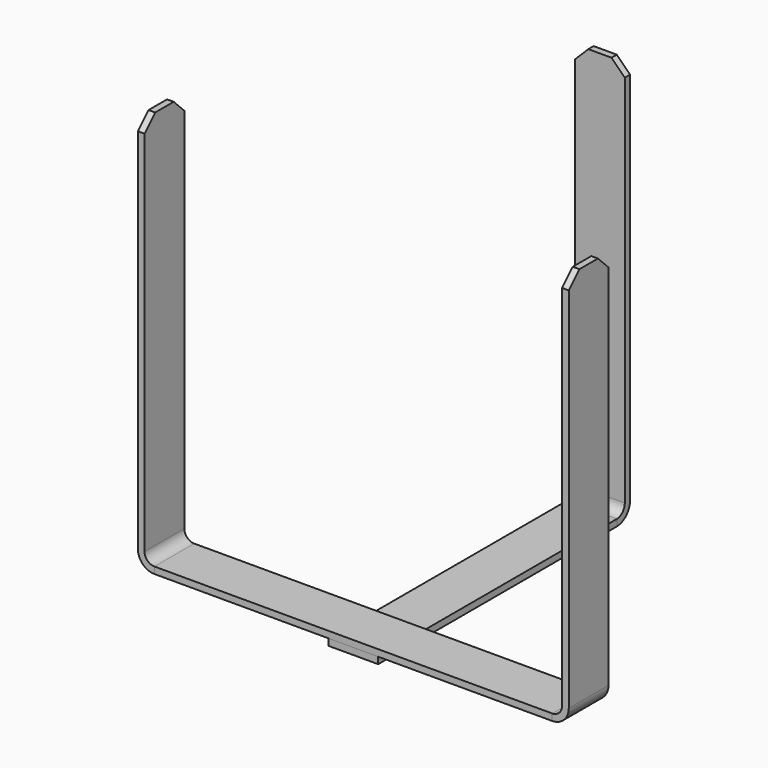
from build123d import *

# Parameters (mm, degrees)
F0_W       = 66.675
F0_H       = 19.05
F8_DEPTH   = 2.54
F0_W_2     = 19.05
F0_H_2     = 95.25
F13_DEPTH  = 2.54
F14_SIZE   = 5.08
F14_2_SIZE = 5.08
F14_3_SIZE = 5.08


with BuildPart() as f4:
    # F4: sweep along a path in F1
    with BuildLine(Plane.XZ) as f4_path:
        Line((82.55, 152.4), (82.55, 6.35))
        ThreePointArc((82.55, 6.35), (80.6901280605, 1.8598719395), (76.2, 0))
    # F3 (on offset) → F4 (sweep)
    with BuildSketch(Plane.YZ.offset(76.2)):
        Polygon((-9.525, 0), (0, 0), (9.525, 0), (9.525, 2.54), (-9.525, 2.54), align=None)
    sweep(path=f4_path.line)

    # F14
    f14_edges = [f4.edges().sort_by_distance(p)[0] for p in [
        (81.28, -9.525, 152.4),
        (81.28, 9.525, 152.4),
    ]]
    chamfer(f14_edges, length=F14_SIZE)


with BuildPart() as f7:
    # F7: sweep along a path in F1
    with BuildLine(Plane.XZ) as f7_path:
        ThreePointArc((-76.2, 0), (-80.6901280605, 1.8598719395), (-82.55, 6.35))
        Line((-82.55, 6.35), (-82.55, 152.4))
    # F6 (on offset) → F7 (sweep)
    with BuildSketch(Plane.YZ.offset(-76.2)):
        Polygon((-9.525, 0), (0, 0), (9.525, 0), (9.525, 2.54), (-9.525, 2.54), align=None)
    sweep(path=f7_path.line)

    # F14#2
    f14_2_edges = [f7.edges().sort_by_distance(p)[0] for p in [
        (-81.28, -9.525, 152.4),
        (-81.28, 9.525, 152.4),
    ]]
    chamfer(f14_2_edges, length=F14_2_SIZE)


with BuildPart() as f8:
    # F0 (on Top) → F8 (new body)
    with BuildSketch(Plane.XY):
        with Locations((42.8625, 0)):
            Rectangle(F0_W, F0_H)
        Polygon((9.525, -9.525), (9.525, 9.525), (-9.525, 9.525), (-9.525, 0), (-9.525, -9.525), align=None)
        Polygon((-9.525, 0), (-9.525, 9.525), (-76.2, 9.525), (-76.2, -9.525), (-9.525, -9.525), align=None)
    extrude(amount=F8_DEPTH)


with BuildPart() as f12:
    # F12: sweep along a path in F11
    with BuildLine(Plane.YZ) as f12_path:
        ThreePointArc((104.775, -2.54), (109.2651280605, -0.6801280605), (111.125, 3.81))
        Line((111.125, 3.81), (111.125, 152.4))
    # F10 (on offset) → F12 (sweep)
    with BuildSketch(Plane.XZ.offset(-104.775)):
        Polygon((9.525, 0), (0, 0), (-9.525, 0), (-9.525, -2.54), (9.525, -2.54), align=None)
    sweep(path=f12_path.line)

    # F14#3
    f14_3_edges = [f12.edges().sort_by_distance(p)[0] for p in [
        (9.525, 109.855, 152.4),
        (-9.525, 109.855, 152.4),
    ]]
    chamfer(f14_3_edges, length=F14_3_SIZE)


with BuildPart() as f13:
    # F0 (on Top) → F13 (new body)
    with BuildSketch(Plane.XY):
        Polygon((9.525, -9.525), (9.525, 9.525), (-9.525, 9.525), (-9.525, 0), (-9.525, -9.525), align=None)
        with Locations((0, 57.15)):
            Rectangle(F0_W_2, F0_H_2)
    extrude(amount=-F13_DEPTH)


solid = Compound([f4.part, f7.part, f8.part, f12.part, f13.part])
